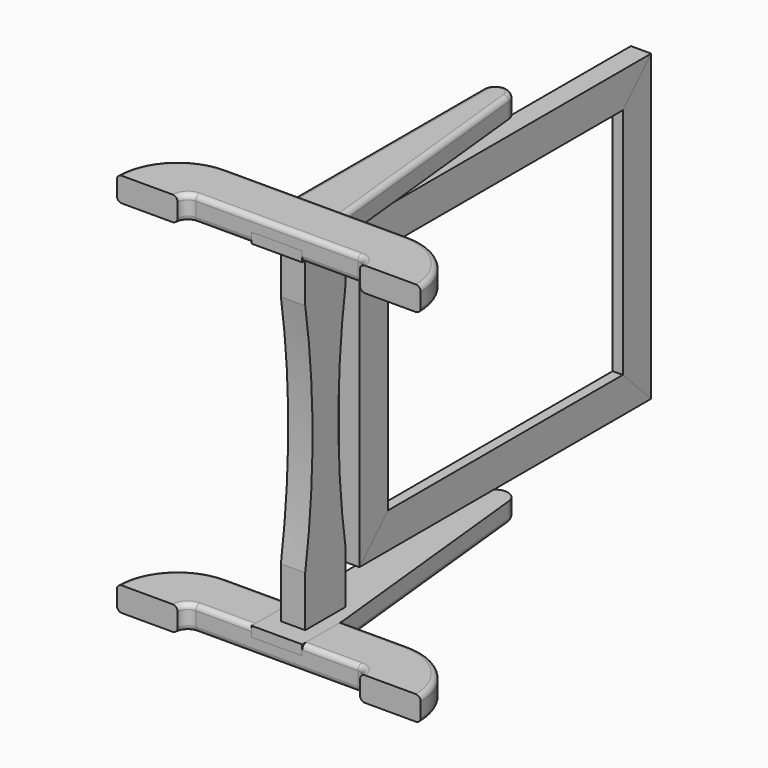
from build123d import *

# Parameters (mm, degrees)
F1_DEPTH  = 24
F2_W      = 50
F2_H      = 10
F3_DEPTH  = 60.001
F4_R      = 5
F6_DEPTH  = 12
F11_DEPTH = 10
F12_DEPTH = 10
F13_DEPTH = 10
F14_DEPTH = 10
F15_DEPTH = 10
F16_DEPTH = 10
F17_DEPTH = 10
F18_DEPTH = 10
F22_DEPTH = 10
F24_DEPTH = 6
F26_DEPTH = 10
F28_DEPTH = 6
F30_DEPTH = 10
F32_DEPTH = 6
F34_DEPTH = 10
F36_DEPTH = 6
F37_W     = 50
F37_H     = 50
F38_DEPTH = 10
F39_DEPTH = 10
F40_W     = 50
F40_H     = 50
F41_DEPTH = 10
F42_R     = 5
F48_DEPTH = 10


with BuildPart() as f1:
    # F0 (on Top) → F1 (new body)
    with BuildSketch(Plane.XY):
        with BuildLine():
            Line((90, -30), (150, -30))
            ThreePointArc((150, -30), (132.4264068712, 12.4264068712), (90, 30))
            Line((90, 30), (-90, 30))
            ThreePointArc((-90, 30), (-132.4264068712, 12.4264068712), (-150, -30))
            Line((-150, -30), (-90, -30))
            ThreePointArc((-90, -30), (-87.0710678119, -22.9289321881), (-80, -20))
            Line((-80, -20), (80, -20))
            ThreePointArc((80, -20), (87.0710678119, -22.9289321881), (90, -30))
        make_face()
    extrude(amount=F1_DEPTH)

    # F2 (on face) → F3 (cut, through all)
    with BuildSketch(Plane(origin=(0, 30, 0), x_dir=(-1, 0, 0), z_dir=(0, 1, 0))):
        with Locations((0, 5)):
            Rectangle(F2_W, F2_H)
    extrude(amount=-F3_DEPTH, mode=Mode.SUBTRACT)

    # F4
    f4_edges = [f1.edges().sort_by_distance(p)[0] for p in [
        (-132.426407, 12.426407, 24),
        (-87.071068, -22.928932, 24),
        (-132.426407, 12.426407, 0),
        (57.5, 30, 0),
        (87.071068, -22.928932, 0),
        (-52.5, -20, 0),
    ]]
    fillet(f4_edges, radius=F4_R)


with BuildPart() as f6:
    # F5 (on Right) → F6 (new body, symmetric)
    with BuildSketch(Plane.YZ):
        with BuildLine():
            Line((29.9430195928, 0), (-20.0569804072, 0))
            Line((-20.0569804073, 0), (-20.0569804073, -50))
            ThreePointArc((-20.0569804073, -50), (-11.0320137248, -166), (-20.0569804073, -282))
            Line((-20.0569804073, -282), (-20.0569804073, -332))
            Line((-20.0569804073, -332), (29.9430195927, -332))
            Line((29.9430195928, -332), (29.9430195928, -282))
            ThreePointArc((29.9430195927, -282), (20.9180529103, -166), (29.9430195927, -50))
            Line((29.9430195928, -50), (29.9430195928, 0))
        make_face()
    extrude(amount=F6_DEPTH, both=True)


with BuildPart() as f6_1:
    # F8: moved
    add(f6.part.moved(Location((0, -100, 0))))


with BuildPart() as f6_2:
    # F9: moved
    add(f6_1.part.moved(Location((0, 120, 0))))


with BuildPart() as f11:
    # F10 (on face) → F11 (new body)
    with BuildSketch(Plane.YZ):
        Polygon((444.9430195928, -16), (409.9430195928, -51), (409.9430195928, -281), (444.9430195928, -316), align=None)
    extrude(amount=F11_DEPTH)

    # F12 (add): a face of the model
    f12_faces = [f11.faces().sort_by_distance(p)[0] for p in [
        (0, 428.2134598443, -166),
    ]]
    extrude(f12_faces, amount=F12_DEPTH)

    # F21 (on face) → F22 (cut)
    with BuildSketch(Plane(origin=(-10, 0, 0), x_dir=(0, -1, 0), z_dir=(-1, 0, 0))):
        Polygon((-419.9430195928, -41), (-419.9430195928, -291), (-409.9430195928, -281), (-409.9430195928, -51), align=None)
    extrude(amount=-F22_DEPTH, mode=Mode.SUBTRACT)

    # F23 (on face) → F24 (cut)
    with BuildSketch(Plane(origin=(-10, 0, 0), x_dir=(0, -1, 0), z_dir=(-1, 0, 0))):
        Polygon((-429.9430195928, -31), (-429.9430195928, -301), (-419.9430195928, -291), (-419.9430195928, -41), align=None)
    extrude(amount=-F24_DEPTH, mode=Mode.SUBTRACT)


with BuildPart() as f13:
    # F10 (on face) → F13 (new body)
    with BuildSketch(Plane.YZ):
        Polygon((119.9430195928, -281), (119.9430195928, -51), (84.9430195928, -16), (84.9430195928, -316), align=None)
    extrude(amount=F13_DEPTH)

    # F14 (add): a face of the model
    f14_faces = [f13.faces().sort_by_distance(p)[0] for p in [
        (0, 101.6725793412, -166),
    ]]
    extrude(f14_faces, amount=F14_DEPTH)

    # F33 (on face) → F34 (cut)
    with BuildSketch(Plane(origin=(-10, 0, 0), x_dir=(0, -1, 0), z_dir=(-1, 0, 0))):
        Polygon((-119.9430195928, -281), (-109.9430195928, -291), (-109.9430195928, -41), (-119.9430195928, -51), align=None)
    extrude(amount=-F34_DEPTH, mode=Mode.SUBTRACT)

    # F35 (on face) → F36 (cut)
    with BuildSketch(Plane(origin=(-10, 0, 0), x_dir=(0, -1, 0), z_dir=(-1, 0, 0))):
        Polygon((-109.9430195928, -291), (-99.9430195928, -301), (-99.9430195928, -31), (-109.9430195928, -41), align=None)
    extrude(amount=-F36_DEPTH, mode=Mode.SUBTRACT)


with BuildPart() as f15:
    # F10 (on face) → F15 (new body)
    with BuildSketch(Plane.YZ):
        Polygon((119.9430195928, -51), (409.9430195928, -51), (444.9430195928, -16), (84.9430195928, -16), align=None)
    extrude(amount=F15_DEPTH)


with BuildPart() as f16:
    # F16 (new): a face of the model
    f16_faces = [f15.part.faces().sort_by_distance(p)[0] for p in [
        (0, 264.9430195928, -32.8717948718),
    ]]
    extrude(f16_faces, amount=F16_DEPTH)

    # F19: union F15
    add(f15.part)

    # F25 (on face) → F26 (cut)
    with BuildSketch(Plane(origin=(-10, 0, 0), x_dir=(0, -1, 0), z_dir=(-1, 0, 0))):
        Polygon((-109.9430195928, -41), (-419.9430195928, -41), (-409.9430195928, -51), (-119.9430195928, -51), align=None)
    extrude(amount=-F26_DEPTH, mode=Mode.SUBTRACT)

    # F27 (on face) → F28 (cut)
    with BuildSketch(Plane(origin=(-10, 0, 0), x_dir=(0, -1, 0), z_dir=(-1, 0, 0))):
        Polygon((-99.9430195928, -31), (-429.9430195928, -31), (-419.9430195928, -41), (-109.9430195928, -41), align=None)
    extrude(amount=-F28_DEPTH, mode=Mode.SUBTRACT)


with BuildPart() as f17:
    # F10 (on face) → F17 (new body)
    with BuildSketch(Plane.YZ):
        Polygon((444.9430195928, -316), (409.9430195928, -281), (119.9430195928, -281), (84.9430195928, -316), align=None)
    extrude(amount=F17_DEPTH)


with BuildPart() as f18:
    # F18 (new): a face of the model
    f18_faces = [f17.part.faces().sort_by_distance(p)[0] for p in [
        (0, 264.9430195928, -299.1282051282),
    ]]
    extrude(f18_faces, amount=F18_DEPTH)


with BuildPart() as f17_1:
    add(f17.part)

    # F20: union F18
    add(f18.part)

    # F29 (on face) → F30 (cut)
    with BuildSketch(Plane(origin=(-10, 0, 0), x_dir=(0, -1, 0), z_dir=(-1, 0, 0))):
        Polygon((-419.9430195928, -291), (-109.9430195928, -291), (-119.9430195928, -281), (-409.9430195928, -281), align=None)
    extrude(amount=-F30_DEPTH, mode=Mode.SUBTRACT)

    # F31 (on face) → F32 (cut)
    with BuildSketch(Plane(origin=(-10, 0, 0), x_dir=(0, -1, 0), z_dir=(-1, 0, 0))):
        Polygon((-429.9430195928, -301), (-99.9430195928, -301), (-109.9430195928, -291), (-419.9430195928, -291), align=None)
    extrude(amount=-F32_DEPTH, mode=Mode.SUBTRACT)


with BuildPart() as f38:
    # F37 (on face) → F38 (new body)
    with BuildSketch(Plane(origin=(0, 0, 10), x_dir=(1, 0, 0), z_dir=(0, 0, -1))):
        with Locations((0, -5)):
            Rectangle(F37_W, F37_H)
        with BuildLine():
            Line((-0.0697488577, -266.3186570972), (25, -30))
            Line((25, -30), (-25, -30))
            Line((-25, -30), (-25, -265))
            ThreePointArc((-25, -265), (-13.1602502259, -277.4825506063), (-0.0697488577, -266.3186570972))
        make_face()
    extrude(amount=F38_DEPTH)

    # F39 (add): a face of the model
    f39_faces = [f38.faces().sort_by_distance(p)[0] for p in [
        (-4.4921738425, 109.3859800759, 10),
    ]]
    extrude(f39_faces, amount=F39_DEPTH)

    # F40 (on face) → F41 (cut)
    with BuildSketch(Plane.XY.offset(20)):
        with Locations((0, 5)):
            Rectangle(F40_W, F40_H)
    extrude(amount=-F41_DEPTH, mode=Mode.SUBTRACT)

    # F42
    f42_edges = [f38.edges().sort_by_distance(p)[0] for p in [
        (12.465126, 148.159329, 20),
        (-13.16025, 277.482551, 20),
        (-25, 147.5, 20),
    ]]
    fillet(f42_edges, radius=F42_R)


with BuildPart() as f43_1:
    # F43: instance of F1
    add(f1.part.mirror(Plane(origin=(-4.4921738425, 109.3859800759, 0), x_dir=(1, 0, 0), z_dir=(0, 0, -1))))


with BuildPart() as f43_2:
    # F43: instance of F38
    add(f38.part.mirror(Plane(origin=(-4.4921738425, 109.3859800759, 0), x_dir=(1, 0, 0), z_dir=(0, 0, -1))))


with BuildPart() as f43_1_1:
    # F44: moved
    add(f43_1.part.moved(Location((0, 0, -332))))


with BuildPart() as f43_2_1:
    # F44: moved
    add(f43_2.part.moved(Location((0, 0, -332))))


with BuildPart() as f11_1:
    # F45: moved
    add(f11.part.moved(Location((0, 0, -0.5))))


with BuildPart() as f17_2:
    # F45: moved
    add(f17_1.part.moved(Location((0, 0, -0.5))))


with BuildPart() as f16_1:
    # F45: moved
    add(f16.part.moved(Location((0, 0, -0.5))))


with BuildPart() as f13_1:
    # F45: moved
    add(f13.part.moved(Location((0, 0, -0.5))))


with BuildPart() as f11_2:
    # F46: moved
    add(f11_1.part.moved(Location((-12.5, 0, 0))))


with BuildPart() as f17_3:
    # F46: moved
    add(f17_2.part.moved(Location((-12.5, 0, 0))))


with BuildPart() as f16_2:
    # F46: moved
    add(f16_1.part.moved(Location((-12.5, 0, 0))))


with BuildPart() as f13_2:
    # F46: moved
    add(f13_1.part.moved(Location((-12.5, 0, 0))))


with BuildPart() as f38_1:
    add(f38.part)

    # F47 (on face) → F48 (cut)
    with BuildSketch(Plane(origin=(0, 0, 0), x_dir=(1, 0, 0), z_dir=(0, 0, -1))):
        with BuildLine():
            Line((-2, -7), (-2, -19))
            ThreePointArc((-2, -19), (0, -21), (2, -19))
            Line((2, -19), (2, -7))
            ThreePointArc((2, -7), (0, -5), (-2, -7))
        make_face()
        with BuildLine():
            Line((-2, -31), (-2, -43))
            ThreePointArc((-2, -43), (0, -45), (2, -43))
            Line((2, -43), (2, -31))
            ThreePointArc((2, -31), (0, -29), (-2, -31))
        make_face()
    extrude(amount=-F48_DEPTH, mode=Mode.SUBTRACT)


solid = Compound([f1.part, f6_2.part, f43_1_1.part, f43_2_1.part, f11_2.part, f17_3.part, f16_2.part, f13_2.part, f38_1.part])
